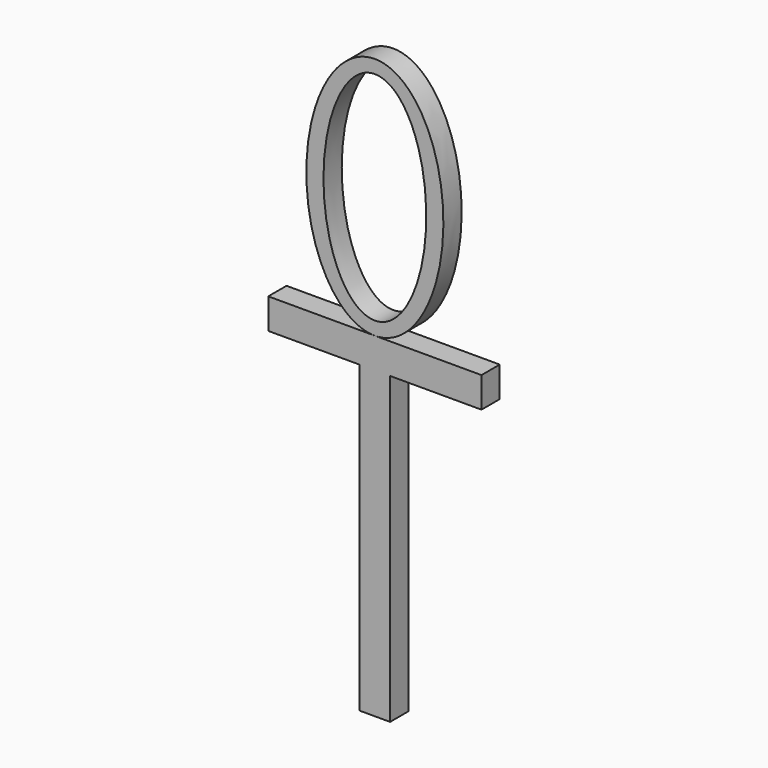
from build123d import *

# Parameters (mm, degrees)
F1_DEPTH = 750


with BuildPart() as f1:
    # F0 (on Front) → F1 (new body)
    with BuildSketch(Plane.XZ):
        with BuildLine():
            add(Edge.make_bspline(
                [(-2750, 12273.3898056417), (-2750, 8273.3898056417), (-500, 8273.3898056417)],
                knots=[1.5707963268, 1.5707963268, 1.5707963268, 3.1415926536, 3.1415926536, 3.1415926536], degree=2, weights=[1, 0.7071067812, 1]))
            Line((-500, 8273.3898056417), (-500, 8710.8898056417))
            add(Edge.make_bspline(
                [(-2187.5, 12273.3898056417), (-2187.5, 8710.8898056417), (-500, 8710.8898056417)],
                knots=[4.7123889804, 4.7123889804, 4.7123889804, 6.2831853072, 6.2831853072, 6.2831853072], degree=2, weights=[1, 0.7071067812, 1]))
            Line((-2187.5, 12273.3898056417), (-2750, 12273.3898056417))
        make_face()
        with BuildLine():
            Line((-500, 8710.8898056417), (-500, 8273.3898056417))
            add(Edge.make_bspline(
                [(-500, 8273.3898056417), (1750, 8273.3898056417), (1750, 12273.3898056417), (1750, 16273.3898056417), (-500, 16273.3898056417)],
                knots=[3.1415926536, 3.1415926536, 3.1415926536, 4.7123889804, 4.7123889804, 6.2831853072, 6.2831853072, 6.2831853072], degree=2, weights=[1, 0.7071067812, 1, 0.7071067812, 1]))
            Line((-500, 16273.3898056417), (-500, 15835.8898056417))
            add(Edge.make_bspline(
                [(-500, 8710.8898056417), (1187.5, 8710.8898056417), (1187.5, 12273.3898056416), (1187.5, 15835.8898056416), (-500, 15835.8898056417)],
                knots=[0, 0, 0, 1.5707963268, 1.5707963268, 3.1415926536, 3.1415926536, 3.1415926536], degree=2, weights=[1, 0.7071067812, 1, 0.7071067812, 1]))
        make_face()
        with BuildLine():
            add(Edge.make_bspline(
                [(-500, 16273.3898056417), (-2750, 16273.3898056417), (-2750, 12273.3898056417)],
                knots=[0, 0, 0, 1.5707963268, 1.5707963268, 1.5707963268], degree=2, weights=[1, 0.7071067812, 1]))
            Line((-2750, 12273.3898056417), (-2187.5, 12273.3898056417))
            add(Edge.make_bspline(
                [(-500, 15835.8898056417), (-2187.5, 15835.8898056417), (-2187.5, 12273.3898056417)],
                knots=[3.1415926536, 3.1415926536, 3.1415926536, 4.7123889804, 4.7123889804, 4.7123889804], degree=2, weights=[1, 0.7071067812, 1]))
            Line((-500, 15835.8898056417), (-500, 16273.3898056417))
        make_face()
    extrude(amount=F1_DEPTH)


with BuildPart() as f1b:
    # F0 (on Front) → F1, piece 2 (new body)
    with BuildSketch(Plane.XZ):
        Polygon((-1000, -2726.6101943583), (0, -2726.6101943583), (0, 7273.3898056417), (3000, 7273.3898056417), (3000, 8273.3898056417), (-500, 8273.3898056417), (-4000, 8273.3898056417), (-4000, 7273.3898056417), (-1000, 7273.3898056417), align=None)
    extrude(amount=F1_DEPTH)


solid = Compound([f1.part, f1b.part])
